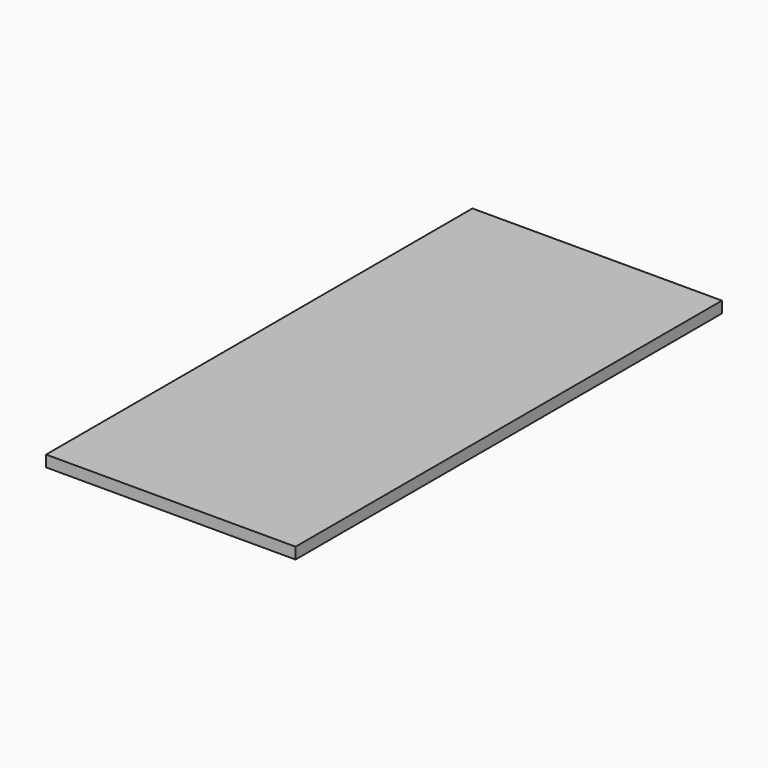
from build123d import *

# Parameters (mm, degrees)
F0_W     = 440
F0_H     = 20
F1_DEPTH = 470
F2_R     = 3
F3_DEPTH = 12
F4_R     = 3
F5_DEPTH = 12
F6_R     = 3
F7_DEPTH = 12
F8_R     = 3
F9_DEPTH = 12


with BuildPart() as f1:
    # F0 (on Front) → F1 (new body, symmetric)
    with BuildSketch(Plane.XZ):
        with Locations((-220, 10)):
            Rectangle(F0_W, F0_H)
    extrude(amount=F1_DEPTH, both=True)

    # F2 (on face) → F3 (cut)
    with BuildSketch(Plane(origin=(0, 0, 0), x_dir=(1, 0, 0), z_dir=(0, 0, -1))):
        with Locations((-400, 420)):
            Circle(F2_R)
    extrude(amount=-F3_DEPTH, mode=Mode.SUBTRACT)

    # F4 (on face) → F5 (cut)
    with BuildSketch(Plane(origin=(0, 0, 0), x_dir=(1, 0, 0), z_dir=(0, 0, -1))):
        with Locations((-40, 420)):
            Circle(F4_R)
    extrude(amount=-F5_DEPTH, mode=Mode.SUBTRACT)

    # F6 (on face) → F7 (cut)
    with BuildSketch(Plane(origin=(0, 0, 0), x_dir=(1, 0, 0), z_dir=(0, 0, -1))):
        with Locations((-400, -420)):
            Circle(F6_R)
    extrude(amount=-F7_DEPTH, mode=Mode.SUBTRACT)

    # F8 (on face) → F9 (cut)
    with BuildSketch(Plane(origin=(0, 0, 0), x_dir=(1, 0, 0), z_dir=(0, 0, -1))):
        with Locations((-40, -420)):
            Circle(F8_R)
    extrude(amount=-F9_DEPTH, mode=Mode.SUBTRACT)


solid = f1.part
